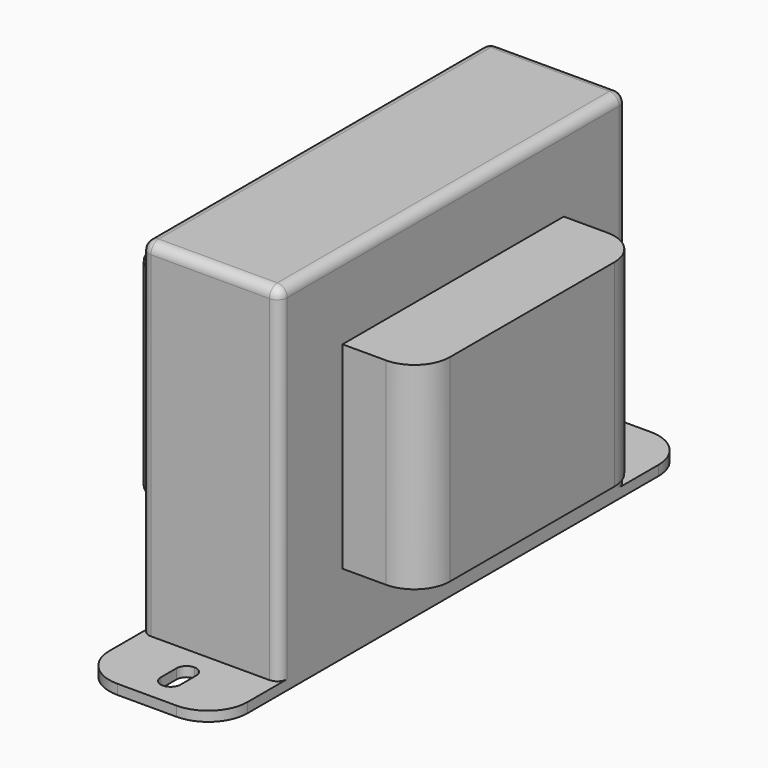
from build123d import *

# Parameters (mm, degrees)
F0_W      = 22.225
F0_H      = 69.85
F1_DEPTH  = 57.15
F2_W      = 22.225
F2_H      = 12.7
F3_DEPTH  = 1.5875
F4_R      = 6.35
F5_W      = 3.175
F5_H      = 6.35
F6_DEPTH  = 25.4
F7_R      = 1.58749
F8_W      = 44.45
F8_H      = 31.75
F10_DEPTH = 12.7
F9_W      = 44.45
F9_H      = 31.75
F11_DEPTH = 12.7
F12_R     = 5.715
F13_R     = 1.5875


# Not quite as in the source:
# - a fillet or chamfer is up to 0.001 mm smaller than in the source, because OpenCascade refuses the exact size


with BuildPart() as f1:
    # F0 (on Top) → F1 (new body)
    with BuildSketch(Plane.XY):
        Rectangle(F0_W, F0_H)
    extrude(amount=F1_DEPTH)

    # F2 (on face) → F3 (join)
    with BuildSketch(Plane(origin=(0, 0, 0), x_dir=(1, 0, 0), z_dir=(0, 0, -1))):
        with Locations((0, 41.275)):
            Rectangle(F2_W, F2_H)
        with Locations((0, -41.275)):
            Rectangle(F2_W, F2_H)
    extrude(amount=-F3_DEPTH)

    # F4
    f4_edges = [f1.edges().sort_by_distance(p)[0] for p in [
        (-11.1125, -47.625, 0.79375),
        (11.1125, -47.625, 0.79375),
        (-11.1125, 47.625, 0.79375),
        (11.1125, 47.625, 0.79375),
    ]]
    fillet(f4_edges, radius=F4_R)

    # F5 (on face) → F6 (cut)
    with BuildSketch(Plane.XY.offset(1.5875)):
        with Locations((0, 41.275)):
            Rectangle(F5_W, F5_H)
        with Locations((0, -41.275)):
            Rectangle(F5_W, F5_H)
    extrude(amount=-F6_DEPTH, mode=Mode.SUBTRACT)

    # F7 (radius 1.5875 in the source; OpenCascade refuses exactly that, so slightly less here)
    f7_edges = [f1.edges().sort_by_distance(p)[0] for p in [
        (1.5875, 44.45, 0.79375),
        (-1.5875, 44.45, 0.79375),
        (-1.5875, 38.1, 0.79375),
        (1.5875, 38.1, 0.79375),
        (1.5875, -38.1, 0.79375),
        (-1.5875, -38.1, 0.79375),
        (-1.5875, -44.45, 0.79375),
        (1.5875, -44.45, 0.79375),
    ]]
    fillet(f7_edges, radius=F7_R)

    # F8 (on face) → F10 (join)
    with BuildSketch(Plane.YZ.offset(11.1125)):
        with Locations((0, 28.575)):
            Rectangle(F8_W, F8_H)
    extrude(amount=F10_DEPTH)

    # F9 (on face) → F11 (join)
    with BuildSketch(Plane(origin=(-11.1125, 0, 0), x_dir=(0, -1, 0), z_dir=(-1, 0, 0))):
        with Locations((0, 28.575)):
            Rectangle(F9_W, F9_H)
    extrude(amount=F11_DEPTH)

    # F12
    f12_edges = [f1.edges().sort_by_distance(p)[0] for p in [
        (23.8125, -22.225, 28.575),
        (23.8125, 22.225, 28.575),
        (-23.8125, -22.225, 28.575),
        (-23.8125, 22.225, 28.575),
    ]]
    fillet(f12_edges, radius=F12_R)

    # F13
    f13_edges = [f1.edges().sort_by_distance(p)[0] for p in [
        (11.1125, -34.925, 29.36875),
        (11.1125, 0, 57.15),
        (11.1125, 34.925, 29.36875),
        (0, -34.925, 57.15),
        (0, 34.925, 57.15),
        (-11.1125, -34.925, 29.36875),
        (-11.1125, 0, 57.15),
        (-11.1125, 34.925, 29.36875),
    ]]
    fillet(f13_edges, radius=F13_R)


solid = f1.part
